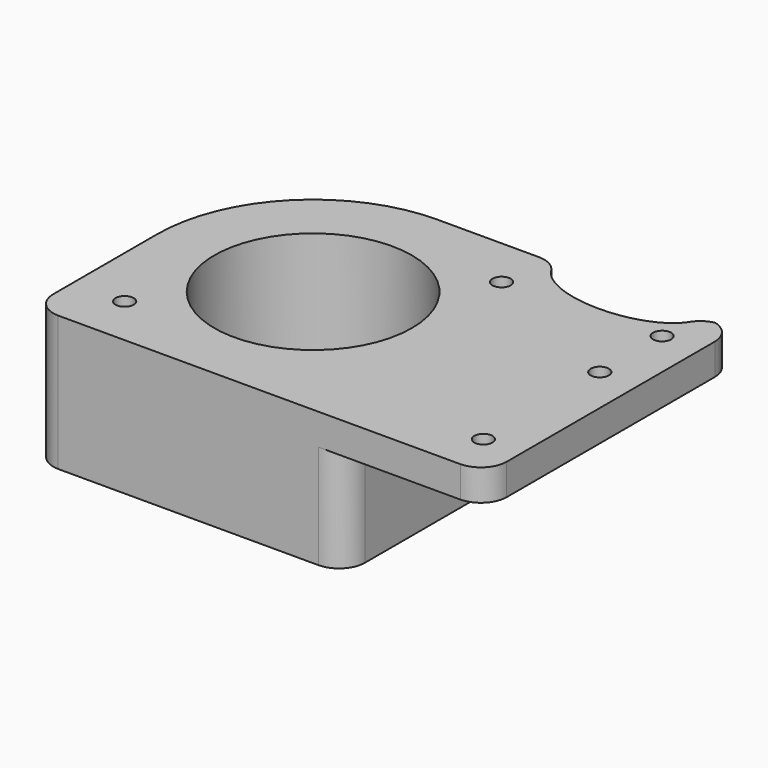
from build123d import *

# Parameters (mm, degrees)
F0_R         = 1.75
F1_DEPTH     = 6
F0_R_2       = 19
F2_DEPTH     = 26
F3_T1_DEPTH  = 51.0048285071
F3_T3_DEPTH  = 32.5024142536
F3_T5_DEPTH  = 23.67798751
F3_T7_DEPTH  = 31.0048285071
F3_T9_DEPTH  = 43.67798751
F3_T11_DEPTH = 28.3837127694


# Not quite as in the source:
# - a fillet or chamfer that OpenCascade refuses, or shapes differently, is made with other operations: its cross-section is extruded or revolved along the edge and cut away or added


with BuildPart() as f1:
    # F0 (on Top) → F1 (new body)
    with BuildSketch(Plane.XY):
        with BuildLine():
            Line((-47.9554124177, 37.5), (-54.25, 37.5))
            add(Edge.make_bspline(
                [(-68.25, 30), (-54.25, 30), (-54.25, 37.5)],
                knots=[1.5707963268, 1.5707963268, 1.5707963268, 3.1415926536, 3.1415926536, 3.1415926536], degree=2, weights=[1, 0.7071067812, 1]))
            Line((-68.25, 30), (-68.25, -22.5))
            Line((-68.25, -22.5), (-47.9554124177, -22.5))
            Line((-47.9554124177, -22.5), (-47.9554124177, 37.5))
        make_face()
        with Locations((-55.2723892033, -14)):
            Circle(F0_R, mode=Mode.SUBTRACT)
        with Locations((-55.2723892033, 13.9999985695)):
            Circle(F0_R, mode=Mode.SUBTRACT)
        with Locations((-55.2723892033, 28.9999985695)):
            Circle(F0_R, mode=Mode.SUBTRACT)
        with BuildLine():
            Line((-68.25, -22.5), (-68.25, 30))
            add(Edge.make_bspline(
                [(-75.25, 31.0048094716), (-72.001288694, 30), (-68.25, 30)],
                knots=[1.0471975512, 1.0471975512, 1.0471975512, 1.5707963268, 1.5707963268, 1.5707963268], degree=2, weights=[1, 0.9659258263, 1]))
            Line((-75.25, 31.0048094716), (-75.25, 30))
            Line((-75.25, 30), (-75.25, -22.5))
            Line((-75.25, -22.5), (-68.25, -22.5))
        make_face()
    extrude(amount=-F1_DEPTH)

    # F0 (on Top) → F2 (join)
    with BuildSketch(Plane.XY):
        with BuildLine():
            add(Edge.make_bspline(
                [(-82.25, 37.5), (-82.25, 33.1698729811), (-75.25, 31.0048094716)],
                knots=[0, 0, 0, 1.0471975512, 1.0471975512, 1.0471975512], degree=2, weights=[1, 0.8660254038, 1]))
            Line((-82.25, 37.5), (-105.25, 37.5))
            ThreePointArc((-105.25, 37.5), (-126.4632034356, 28.7132034356), (-135.25, 7.5))
            Line((-135.25, 7.5), (-135.25, -22.5))
            Line((-135.25, -22.5), (-75.25, -22.5))
            Line((-75.25, -22.5), (-75.25, 30))
            Line((-75.25, 30), (-75.25, 31.0048094716))
        make_face()
        with Locations((-125.4025432638, -12.6525432638)):
            Circle(F0_R, mode=Mode.SUBTRACT)
        with Locations((-105.25, 7.5)):
            Circle(F0_R_2, mode=Mode.SUBTRACT)
        with Locations((-85.0974567362, 27.6525432638)):
            Circle(F0_R, mode=Mode.SUBTRACT)
    extrude(amount=-F2_DEPTH)

    # F3: fillet of radius 5 on 8 edges, made by hand

    # F3_s2 → F3_t1 (cut)
    with BuildSketch(Plane.XY.offset(-38.5024142536)):
        with BuildLine():
            ThreePointArc((-130.2490343146, -22.5004), (-133.7855339059, -21.0355339059), (-135.2504, -17.4990343146))
            Line((-135.2504, -17.4990343146), (-135.7505365685, -17.4990343146))
            ThreePointArc((-135.7505365685, -17.4990343146), (-135.7501365685, -19.9995171573), (-135.7501365685, -22.5))
            Line((-135.7501365685, -22.5), (-135.25, -23.0001365685))
            ThreePointArc((-135.25, -23.0001365685), (-132.7495171573, -23.0001365685), (-130.2490343146, -23.0005365685))
            Line((-130.2490343146, -23.0005365685), (-130.2490343146, -22.5004))
        make_face()
    extrude(amount=F3_T1_DEPTH, mode=Mode.SUBTRACT)

    # F3_s4 → F3_t3 (cut)
    with BuildSketch(Plane.XY.offset(-38.5024142536)):
        with BuildLine():
            ThreePointArc((-80.2509656854, -22.5004), (-76.7144660941, -21.0355339059), (-75.2496, -17.4990343146))
            Line((-75.2496, -17.4990343146), (-74.7494634315, -17.4990343146))
            ThreePointArc((-74.7494634315, -17.4990343146), (-74.7498634315, -19.9995171573), (-74.7498634315, -22.5))
            Line((-74.7498634315, -22.5), (-75.25, -23.0001365685))
            ThreePointArc((-75.25, -23.0001365685), (-77.7504828427, -23.0001365685), (-80.2509656854, -23.0005365685))
            Line((-80.2509656854, -23.0005365685), (-80.2509656854, -22.5004))
        make_face()
    extrude(amount=F3_T3_DEPTH, mode=Mode.SUBTRACT)

    # F3_s6 → F3_t5 (cut)
    with BuildSketch(Plane.XY.offset(-14.838993755)):
        with BuildLine():
            ThreePointArc((-50.7144025206, 37.5004), (-53.1463779594, 36.8692922228), (-54.9645855955, 35.1352441979))
            Line((-54.9645855955, 35.1352441979), (-55.389603903, 35.3988651863))
            ThreePointArc((-55.389603903, 35.3988651863), (-54.9183796159, 36.414502766), (-54.7501365685, 37.5))
            Line((-54.7501365685, 37.5), (-54.25, 38.0001365685))
            ThreePointArc((-54.25, 38.0001365685), (-52.4822012603, 38.0001365685), (-50.7144025206, 38.0005365685))
            Line((-50.7144025206, 38.0005365685), (-50.7144025206, 37.5004))
        make_face()
    extrude(amount=F3_T5_DEPTH, mode=Mode.SUBTRACT)

    # F3_s8 → F3_t7 (cut)
    with BuildSketch(Plane.XY.offset(-18.5024142536)):
        with BuildLine():
            ThreePointArc((-52.9563781031, 37.5004), (-49.4198785117, 36.0355339059), (-47.9550124177, 32.4990343146))
            Line((-47.9550124177, 32.4990343146), (-47.4548758491, 32.4990343146))
            ThreePointArc((-47.4548758491, 32.4990343146), (-47.4552758491, 34.9995171573), (-47.4552758491, 37.5))
            Line((-47.4552758491, 37.5), (-47.9554124177, 38.0001365685))
            ThreePointArc((-47.9554124177, 38.0001365685), (-50.4558952604, 38.0001365685), (-52.9563781031, 38.0005365685))
            Line((-52.9563781031, 38.0005365685), (-52.9563781031, 37.5004))
        make_face()
        with BuildLine():
            ThreePointArc((-52.9563781031, -22.5004), (-49.4198785117, -21.0355339059), (-47.9550124177, -17.4990343146))
            Line((-47.9550124177, -17.4990343146), (-47.4548758491, -17.4990343146))
            ThreePointArc((-47.4548758491, -17.4990343146), (-47.4552758491, -19.9995171573), (-47.4552758491, -22.5))
            Line((-47.4552758491, -22.5), (-47.9554124177, -23.0001365685))
            ThreePointArc((-47.9554124177, -23.0001365685), (-50.4558952604, -23.0001365685), (-52.9563781031, -23.0005365685))
            Line((-52.9563781031, -23.0005365685), (-52.9563781031, -22.5004))
        make_face()
    extrude(amount=F3_T7_DEPTH, mode=Mode.SUBTRACT)

    # F3_s10 → F3_t9 (cut)
    with BuildSketch(Plane.XY.offset(-34.838993755)):
        with BuildLine():
            ThreePointArc((-81.5354144045, 35.1352441979), (-83.3536220406, 36.8692922228), (-85.7855974794, 37.5004))
            Line((-85.7855974794, 37.5004), (-85.7855974794, 38.0005365685))
            ThreePointArc((-85.7855974794, 38.0005365685), (-84.0177987397, 38.0001365685), (-82.25, 38.0001365685))
            Line((-82.25, 38.0001365685), (-81.7498634315, 37.5))
            ThreePointArc((-81.7498634315, 37.5), (-81.5816203841, 36.414502766), (-81.110396097, 35.3988651863))
            Line((-81.110396097, 35.3988651863), (-81.5354144045, 35.1352441979))
        make_face()
    extrude(amount=F3_T9_DEPTH, mode=Mode.SUBTRACT)

    # F3_s12 → F3_t11 (cut)
    with BuildSketch(Plane.XY.offset(-34.3837127694)):
        with BuildLine():
            ThreePointArc((-77.9590299164, 32.0970407857), (-75.9803326171, 30.2544669483), (-75.2496, 27.6513243877))
            Line((-75.2496, 27.6513243877), (-74.7493950565, 27.6513243877))
            ThreePointArc((-74.7493950565, 27.6513243877), (-74.7497950565, 29.3280669297), (-74.7497950565, 31.0048094716))
            Line((-74.7497950565, 31.0048094716), (-75.1021974152, 31.4826790996))
            ThreePointArc((-75.1021974152, 31.4826790996), (-76.4425248665, 31.9557259843), (-77.7297679646, 32.5416124255))
            Line((-77.7297679646, 32.5416124255), (-77.9590299164, 32.0970407857))
        make_face()
    extrude(amount=F3_T11_DEPTH, mode=Mode.SUBTRACT)


solid = f1.part
